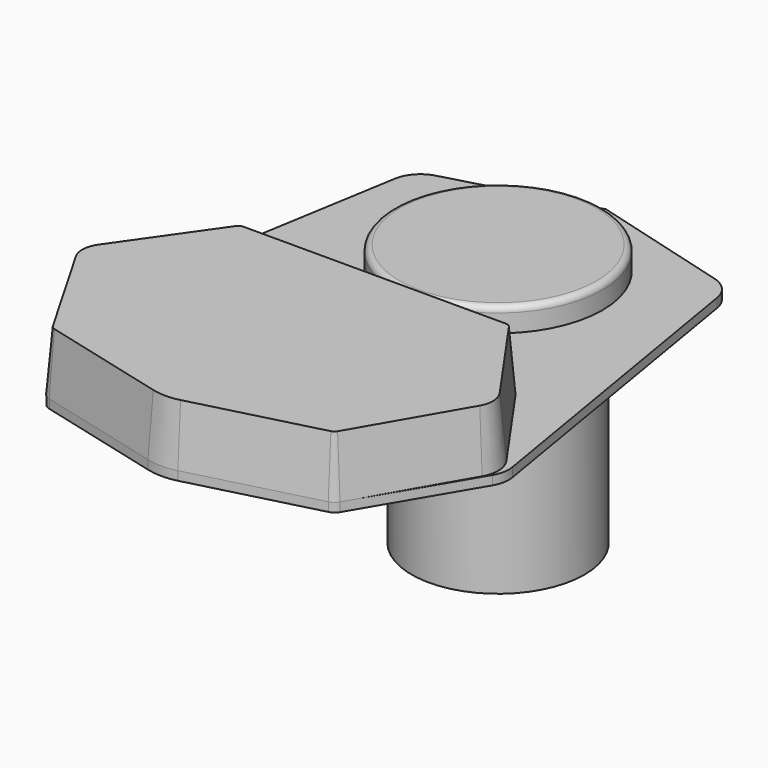
from build123d import *

# Parameters (mm, degrees)
F1_DEPTH  = 10
F1_TAPER  = 5
F2_R      = 6.5
F2_R_2    = 2
F3_DEPTH  = 1
F4_R      = 17.5
F5_DEPTH  = 4
F6_R      = 1
F7_R      = 14.5
F8_DEPTH  = 40
F9_R      = 6.5
F9_R_2    = 15
F10_DEPTH = 1.524


with BuildPart() as f1:
    # F0 (on Top) → F1 (new body)
    with BuildSketch(Plane.XY):
        with BuildLine():
            Line((21.9702988723, 0), (0, 0))
            Line((0, 0), (-21.9702988723, 0))
            ThreePointArc((-21.9702988723, 0), (-22.8937960987, -0.2259783336), (-23.6086029609, -0.8528471273))
            Line((-23.6086029609, -0.8528471273), (-34.37664856, -16.2312099862))
            ThreePointArc((-34.37664856, -16.2312099862), (-35.2761294464, -18.8809952311), (-34.6110153574, -21.5990921679))
            Line((-34.6110153574, -21.5990921679), (-24.6230258112, -38.8987975274))
            ThreePointArc((-24.6230258112, -38.8987975274), (-24.1015629797, -39.4908015325), (-23.3917350118, -39.8350928082))
            Line((-23.3917350118, -39.8350928082), (-2.5038000405, -45.2370800926))
            ThreePointArc((-2.5038000405, -45.2370800926), (0, -45.5556036889), (2.5038000405, -45.2370800926))
            Line((2.5038000405, -45.2370800926), (23.3917350118, -39.8350928082))
            ThreePointArc((23.3917350118, -39.8350928082), (24.1015629797, -39.4908015325), (24.6230258112, -38.8987975274))
            Line((24.6230258112, -38.8987975274), (34.6110153574, -21.5990921679))
            ThreePointArc((34.6110153574, -21.5990921679), (35.2761294464, -18.8809952311), (34.37664856, -16.2312099862))
            Line((34.37664856, -16.2312099862), (23.6086029609, -0.8528471273))
            ThreePointArc((23.6086029609, -0.8528471273), (22.8937960987, -0.2259783336), (21.9702988723, 0))
        make_face()
    extrude(amount=F1_DEPTH, taper=F1_TAPER)

    # F2 (on face) → F3 (join)
    with BuildSketch(Plane(origin=(0, 0, 0), x_dir=(1, 0, 0), z_dir=(0, 0, -1))):
        with Locations((-27.5, 18.8809952311)):
            Circle(F2_R)
        with Locations((-27.5, 18.8809952311)):
            Circle(F2_R_2, mode=Mode.SUBTRACT)
        with Locations((27.5, 18.8809952311)):
            Circle(F2_R)
        with Locations((27.5, 18.8809952311)):
            Circle(F2_R_2, mode=Mode.SUBTRACT)
    extrude(amount=F3_DEPTH)


with BuildPart() as f5:
    # F4 (on Top) → F5 (new body)
    with BuildSketch(Plane.XY):
        with Locations((0, 25)):
            Circle(F4_R)
    extrude(amount=F5_DEPTH)

    # F6
    f6_edges = [f5.edges().sort_by_distance(p)[0] for p in [
        (-17.5, 25, 4),
    ]]
    fillet(f6_edges, radius=F6_R)

    # F7 (on face) → F8 (join)
    with BuildSketch(Plane(origin=(0, 0, 0), x_dir=(1, 0, 0), z_dir=(0, 0, -1))):
        with Locations((0, -25)):
            Circle(F7_R)
    extrude(amount=F8_DEPTH)


with BuildPart() as f10:
    # F9 (on Top) → F10 (new body)
    with BuildSketch(Plane.XY):
        with BuildLine():
            ThreePointArc((-36.0842868047, -17.0996168992), (-36.069131089, -18.8360325364), (-35.4610002497, -20.4625459372))
            Line((-35.4610002497, -20.4625459372), (-24.6241585752, -38.8597979669))
            ThreePointArc((-24.6241585752, -38.8597979669), (-24.1045295476, -39.441991589), (-23.401659071, -39.7810149406))
            Line((-23.401659071, -39.7810149406), (-2.5037875188, -45.1855431631))
            ThreePointArc((-2.5037875188, -45.1855431631), (0, -45.504063521), (2.5037875188, -45.1855431631))
            Line((2.5037875188, -45.1855431631), (23.401659071, -39.7810149406))
            ThreePointArc((23.401659071, -39.7810149406), (24.1045295476, -39.441991589), (24.6241585752, -38.8597979669))
            Line((24.6241585752, -38.8597979669), (35.4610002497, -20.4625459372))
            ThreePointArc((35.4610002497, -20.4625459372), (36.069131089, -18.8360325364), (36.0842868047, -17.0996168992))
            Line((36.0842868047, -17.0996168992), (27.0075972916, 37.1409717984))
            ThreePointArc((27.0075972916, 37.1409717984), (25.7918966711, 39.6613883732), (23.4123663286, 41.1338906851))
            Line((23.4123663286, 41.1338906851), (0, 47.6267471122))
            Line((0, 47.6267471122), (-23.4123663286, 41.1338906851))
            ThreePointArc((-23.4123663286, 41.1338906851), (-25.7918966711, 39.6613883732), (-27.0075972916, 37.1409717984))
            Line((-27.0075972916, 37.1409717984), (-36.0842868047, -17.0996168992))
        make_face()
        with Locations((-27.5, -18.8809952311)):
            Circle(F9_R, mode=Mode.SUBTRACT)
        with Locations((27.5, -18.8809952311)):
            Circle(F9_R, mode=Mode.SUBTRACT)
        with Locations((0, 25)):
            Circle(F9_R_2, mode=Mode.SUBTRACT)
    extrude(amount=-F10_DEPTH)


solid = Compound([f1.part, f5.part, f10.part])
